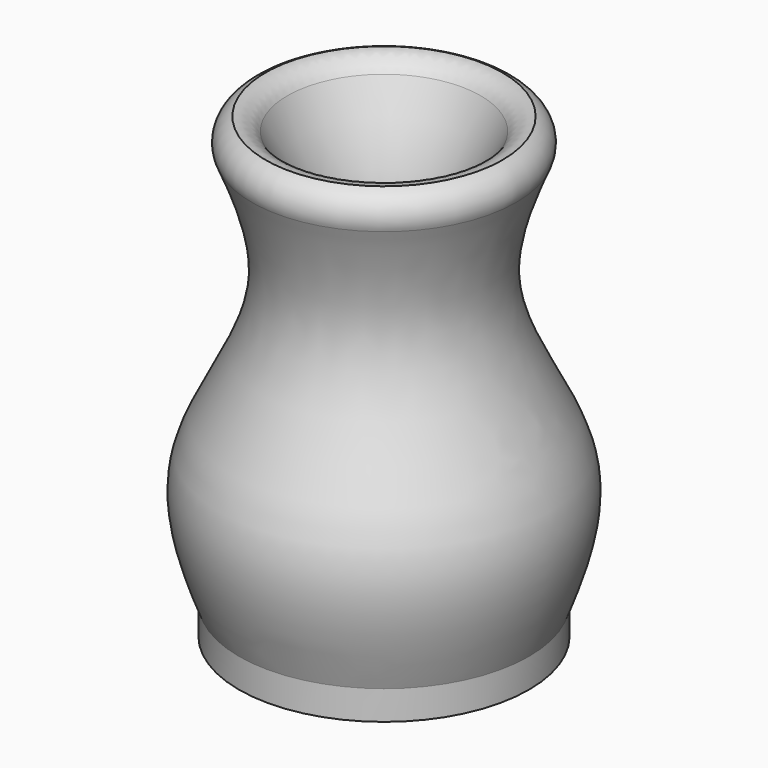
from build123d import *

# Parameters (mm, degrees)
F2_R = 3.81


# Not quite as in the source:
# - a fillet or chamfer that OpenCascade refuses, or shapes differently, is made with other operations: its cross-section is extruded or revolved along the edge and cut away or added


with BuildPart() as f1:
    # F0 (on Front) → F1 (revolve)
    with BuildSketch(Plane.XZ):
        with BuildLine():
            Line((16.0311479121, 4.5178690925), (22.4436055869, 4.5178690925))
            add(Edge.make_bspline(
                [(22.4436055869, 4.5178690925), (24.8600250445, 11.0818898502), (30.0796146771, 25.2605104483), (9.8862561783, 47.130113274), (22.5218644375, 69.4640848416), (22.5048259424, 70.7529232387), (22.4827266771, 70.8515682757)],
                knots=[0, 0, 0, 0, 0.2969827086, 0.6414978418, 0.9493958447, 0.9840559336, 0.9840559336, 0.9840559336, 0.9840559336], degree=3))
            Line((22.4827266771, 70.8515682757), (16.0311479121, 70.8515682757))
            add(Edge.make_bspline(
                [(16.0311479121, 70.8515682757), (12.2960300416, 63.7655309581), (4.4341449473, 48.8504431093), (25.6194031292, 24.2310595898), (19.0460076919, 10.7163383464), (16.0311479121, 4.5178690925)],
                knots=[0, 0, 0, 0, 0.3288488059, 0.6921793675, 1, 1, 1, 1], degree=3))
        make_face()
        Polygon((0, 4.5178690925), (0, 0), (22.4436055869, 0), (22.4436055869, 4.5178690925), (16.0311479121, 4.5178690925), align=None)
    revolve(axis=Axis((0, 0, 38.2318794727), (0, 0, 1)))

    # F2
    f2_edges = [f1.edges().sort_by_distance(p)[0] for p in [
        (-16.031148, 0, 70.851568),
    ]]
    fillet(f2_edges, radius=F2_R)

    # F3: fillet of radius 3.81 on 1 edges, made by hand

    # F3_s1 → F3_t2 (revolve, cut)
    with BuildSketch(Plane.XZ):
        with BuildLine():
            ThreePointArc((18.3344840685, 70.8515682757), (20.4893461193, 68.7718326579), (20.4753256974, 65.7770815621))
            Line((20.4753256974, 65.7770815621), (20.5452530272, 65.7468060184))
            ThreePointArc((20.5452530272, 65.7468060184), (21.6482045261, 68.2389620465), (22.5570835846, 70.8682263162))
            Line((22.5570835846, 70.8682263162), (22.4827266771, 70.9277682757))
            ThreePointArc((22.4827266771, 70.9277682757), (20.4086053728, 70.9277682757), (18.3615945657, 70.9227824663))
            Line((18.3615945657, 70.9227824663), (18.3344840685, 70.8515682757))
        make_face()
    revolve(axis=Axis((0, 0, 70.8515682757), (0, 0, 1)), mode=Mode.SUBTRACT)


solid = f1.part
